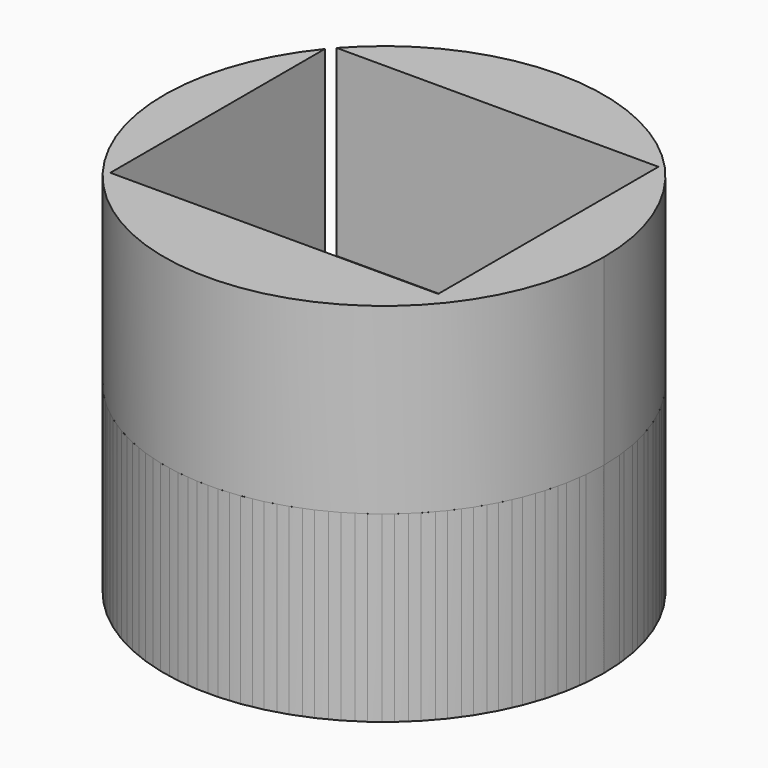
from build123d import *

# Parameters (mm, degrees)
F0_R     = 30
F2_DEPTH = 25
F3_DEPTH = 25


with BuildPart() as f2:
    # F0 (on Top) → F2 (new body)
    with BuildSketch(Plane.XY):
        Circle(F0_R)
    extrude(amount=-F2_DEPTH)


with BuildPart() as f2b:
    # F1 (on face) → F2, piece 2 (new body)
    with BuildSketch(Plane.XY):
        with BuildLine():
            ThreePointArc((30, 0), (10.6658995578, 28.0399462664), (-22.4159057749, 19.9380833656))
            Line((-22.4159057749, 19.9380833656), (21.5137880296, 19.9380833656))
            Line((21.5137880296, 19.9380833656), (21.5137880296, -17.6452174783))
            Line((21.5137880296, -17.6452174783), (-23.2494380325, -17.6452174783))
            Line((-23.2494380325, -17.6452174783), (-23.2494380325, 18.9595261326))
            ThreePointArc((-23.2494380325, 18.9595261326), (-10.0627247559, -28.262016391), (30, 0))
        make_face()
    extrude(amount=-F2_DEPTH)


with BuildPart() as f3:
    # F3 (new): a face of the model
    f3_faces = [f2b.part.faces().sort_by_distance(p)[0] for p in [
        (-9.7781079194, -27.4626458534, 0),
    ]]
    extrude(f3_faces, amount=F3_DEPTH)


solid = Compound([f2.part, f2b.part, f3.part])
